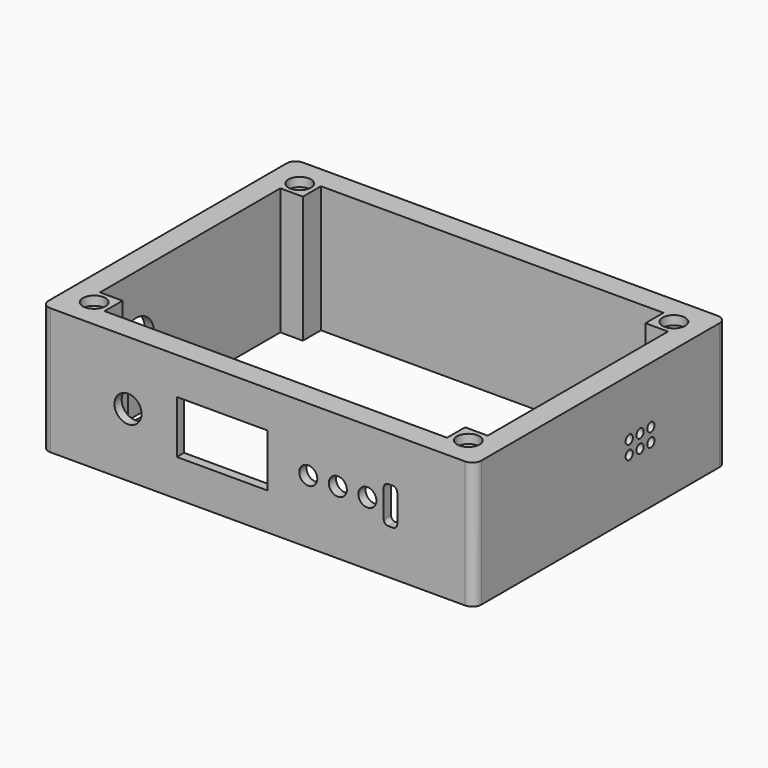
from build123d import *

# Parameters (mm, degrees)
F1_DEPTH  = 28.136
F3_R      = 2.5
F4_DEPTH  = 2
F5_W      = 5
F5_H      = 50
F5_W_2    = 76
F5_H_2    = 5
F6_DEPTH  = 28.137
F7_R      = 1
F8_DEPTH  = 5
F9_R      = 11.25
F9_R_2    = 5
F10_DEPTH = 3
F11_DEPTH = 5
F12_W     = 20.16
F12_H     = 11.72
F12_R     = 3
F12_R_2   = 2
F13_DEPTH = 5
F12_W_2   = 66
F12_H_2   = 18
F12_R_3   = 1.8
F14_DEPTH = 3
F15_DEPTH = 3
F12_R_4   = 0.8
F16_DEPTH = 1.9
F17_DEPTH = 1.9
F18_DEPTH = 1.9
F19_R     = 2.5
F20_DEPTH = 2


# Not quite as in the source:
# - a feature names something its author has since deleted; it is built from what else it names


with BuildPart() as f1:
    # F0 (on Top) → F1 (new body)
    with BuildSketch(Plane.XY):
        with BuildLine():
            Line((46, 35), (-46, 35))
            ThreePointArc((-46, 35), (-47.4142135624, 34.4142135624), (-48, 33))
            Line((-48, 33), (-48, -33))
            ThreePointArc((-48, -33), (-47.4142135624, -34.4142135624), (-46, -35))
            Line((-46, -35), (46, -35))
            ThreePointArc((46, -35), (47.4142135624, -34.4142135624), (48, -33))
            Line((48, -33), (48, 33))
            ThreePointArc((48, 33), (47.4142135624, 34.4142135624), (46, 35))
        make_face()
    extrude(amount=F1_DEPTH)

    # F3 (on face) → F4 (cut)
    with BuildSketch(Plane(origin=(0, 0, 0), x_dir=(1, 0, 0), z_dir=(0, 0, -1))):
        with Locations((-41.5, -28.5)):
            Circle(F3_R)
        with Locations((-41.4999984205, 28.5)):
            Circle(F3_R)
        with Locations((41.5, 28.5)):
            Circle(F3_R)
        with Locations((41.5, -28.5)):
            Circle(F3_R)
    extrude(amount=-F4_DEPTH, mode=Mode.SUBTRACT)

    # F5 (on face) → F6 (cut, through all)
    with BuildSketch(Plane.XY.offset(28.136)):
        with Locations((-40.5, 0)):
            Rectangle(F5_W, F5_H)
        with Locations((0, -27.5)):
            Rectangle(F5_W_2, F5_H_2)
        Rectangle(F5_W_2, F5_H)
        with Locations((0, 27.5)):
            Rectangle(F5_W_2, F5_H_2)
        with Locations((40.5, 0)):
            Rectangle(F5_W, F5_H)
    extrude(amount=-F6_DEPTH, mode=Mode.SUBTRACT)

    # F7 (on face) → F8 (cut, through all)
    with BuildSketch(Plane.YZ.offset(48)):
        with Locations((7.9999985173, 15.568)):
            Circle(F7_R)
        with Locations((7.9999985173, 12.568)):
            Circle(F7_R)
        with Locations((10.9999985173, 12.568)):
            Circle(F7_R)
        with Locations((10.9999985173, 15.568)):
            Circle(F7_R)
        with Locations((13.9999985173, 15.568)):
            Circle(F7_R)
        with Locations((13.9999985173, 12.568)):
            Circle(F7_R)
    extrude(amount=-F8_DEPTH, mode=Mode.SUBTRACT)

    # F9 (on face) → F10 (cut)
    with BuildSketch(Plane(origin=(-48, 0, 0), x_dir=(0, -1, 0), z_dir=(-1, 0, 0))):
        with Locations((15, 14.068)):
            Circle(F9_R)
        with Locations((15, 14.068)):
            Circle(F9_R_2, mode=Mode.SUBTRACT)
    extrude(amount=-F10_DEPTH, mode=Mode.SUBTRACT)

    # F9 (on face) → F11 (cut, through all)
    with BuildSketch(Plane(origin=(-48, 0, 0), x_dir=(0, -1, 0), z_dir=(-1, 0, 0))):
        with Locations((15, 14.068)):
            Circle(F9_R_2)
    extrude(amount=-F11_DEPTH, mode=Mode.SUBTRACT)

    # F12 (on face) → F13 (cut, through all)
    with BuildSketch(Plane(origin=(0, -30, 0), x_dir=(-1, 0, 0), z_dir=(0, 1, 0))):
        with Locations((7.8799169147, 14.0678631142)):
            Rectangle(F12_W, F12_H)
        with Locations((28.7899169147, 14.0678631142)):
            Circle(F12_R)
        with Locations((-11.2000830853, 14.0678631142)):
            Circle(F12_R_2)
        with Locations((-17.7600830853, 14.0678631142)):
            Circle(F12_R_2)
        with Locations((-24.3100830853, 14.0678631142)):
            Circle(F12_R_2)
        with BuildLine():
            ThreePointArc((-30.9400830853, 10.9678631142), (-30.6471898665, 10.260756333), (-29.9400830853, 9.9678631142))
            Line((-29.9400830853, 9.9678631142), (-28.9400830853, 9.9678631142))
            ThreePointArc((-28.9400830853, 9.9678631142), (-28.2329763041, 10.260756333), (-27.9400830853, 10.9678631142))
            Line((-27.9400830853, 10.9678631142), (-27.9400830853, 17.1678631142))
            ThreePointArc((-27.9400830853, 17.1678631142), (-28.2329763041, 17.8749698954), (-28.9400830853, 18.1678631142))
            Line((-28.9400830853, 18.1678631142), (-29.9400830853, 18.1678631142))
            ThreePointArc((-29.9400830853, 18.1678631142), (-30.6471898665, 17.8749698954), (-30.9400830853, 17.1678631142))
            Line((-30.9400830853, 17.1678631142), (-30.9400830853, 10.9678631142))
        make_face()
    extrude(amount=-F13_DEPTH, mode=Mode.SUBTRACT)

    # F12 (on face) → F14 (cut)
    with BuildSketch(Plane(origin=(0, -30, 0), x_dir=(-1, 0, 0), z_dir=(0, 1, 0))):
        with Locations((-0.2100830853, 14.0678631142)):
            Rectangle(F12_W_2, F12_H_2)
        with BuildLine():
            Line((-28.9400830853, 9.9678631142), (-29.9400830853, 9.9678631142))
            ThreePointArc((-29.9400830853, 9.9678631142), (-30.6471898665, 10.260756333), (-30.9400830853, 10.9678631142))
            Line((-30.9400830853, 10.9678631142), (-30.9400830853, 17.1678631142))
            ThreePointArc((-30.9400830853, 17.1678631142), (-30.6471898665, 17.8749698954), (-29.9400830853, 18.1678631142))
            Line((-29.9400830853, 18.1678631142), (-28.9400830853, 18.1678631142))
            ThreePointArc((-28.9400830853, 18.1678631142), (-28.2329763041, 17.8749698954), (-27.9400830853, 17.1678631142))
            Line((-27.9400830853, 17.1678631142), (-27.9400830853, 10.9678631142))
            ThreePointArc((-27.9400830853, 10.9678631142), (-28.2329763041, 10.260756333), (-28.9400830853, 9.9678631142))
        make_face(mode=Mode.SUBTRACT)
        with Locations((-24.3100830853, 14.0678631142)):
            Circle(F12_R_2, mode=Mode.SUBTRACT)
        with Locations((-17.7600830853, 14.0678631142)):
            Circle(F12_R_2, mode=Mode.SUBTRACT)
        with Locations((-11.2000830853, 14.0678631142)):
            Circle(F12_R_2, mode=Mode.SUBTRACT)
        with Locations((7.8799169147, 14.0678631142)):
            Rectangle(F12_W, F12_H, mode=Mode.SUBTRACT)
        with Locations((30.1299169147, 7.5678631142)):
            Circle(F12_R_3, mode=Mode.SUBTRACT)
        with Locations((28.7899169147, 14.0678631142)):
            Circle(F12_R, mode=Mode.SUBTRACT)
        with Locations((-24.0500830853, 20.5678631142)):
            Circle(F12_R_3, mode=Mode.SUBTRACT)
        with Locations((30.1299169147, 20.5678631142)):
            Circle(F12_R_3, mode=Mode.SUBTRACT)
    extrude(amount=F14_DEPTH, mode=Mode.SUBTRACT)

    # F12 (on face) → F15 (cut)
    with BuildSketch(Plane(origin=(0, -30, 0), x_dir=(-1, 0, 0), z_dir=(0, 1, 0))):
        with Locations((-0.2100830853, 14.0678631142)):
            Rectangle(F12_W_2, F12_H_2)
        with BuildLine():
            Line((-28.9400830853, 9.9678631142), (-29.9400830853, 9.9678631142))
            ThreePointArc((-29.9400830853, 9.9678631142), (-30.6471898665, 10.260756333), (-30.9400830853, 10.9678631142))
            Line((-30.9400830853, 10.9678631142), (-30.9400830853, 17.1678631142))
            ThreePointArc((-30.9400830853, 17.1678631142), (-30.6471898665, 17.8749698954), (-29.9400830853, 18.1678631142))
            Line((-29.9400830853, 18.1678631142), (-28.9400830853, 18.1678631142))
            ThreePointArc((-28.9400830853, 18.1678631142), (-28.2329763041, 17.8749698954), (-27.9400830853, 17.1678631142))
            Line((-27.9400830853, 17.1678631142), (-27.9400830853, 10.9678631142))
            ThreePointArc((-27.9400830853, 10.9678631142), (-28.2329763041, 10.260756333), (-28.9400830853, 9.9678631142))
        make_face(mode=Mode.SUBTRACT)
        with Locations((-24.3100830853, 14.0678631142)):
            Circle(F12_R_2, mode=Mode.SUBTRACT)
        with Locations((-17.7600830853, 14.0678631142)):
            Circle(F12_R_2, mode=Mode.SUBTRACT)
        with Locations((-11.2000830853, 14.0678631142)):
            Circle(F12_R_2, mode=Mode.SUBTRACT)
        with Locations((7.8799169147, 14.0678631142)):
            Rectangle(F12_W, F12_H, mode=Mode.SUBTRACT)
        with Locations((30.1299169147, 7.5678631142)):
            Circle(F12_R_3, mode=Mode.SUBTRACT)
        with Locations((28.7899169147, 14.0678631142)):
            Circle(F12_R, mode=Mode.SUBTRACT)
        with Locations((-24.0500830853, 20.5678631142)):
            Circle(F12_R_3, mode=Mode.SUBTRACT)
        with Locations((30.1299169147, 20.5678631142)):
            Circle(F12_R_3, mode=Mode.SUBTRACT)
    extrude(amount=-F15_DEPTH, mode=Mode.SUBTRACT)

    # F12 (on face) → F16 (join)
    with BuildSketch(Plane(origin=(0, -30, 0), x_dir=(-1, 0, 0), z_dir=(0, 1, 0))):
        with Locations((30.1299169147, 20.5678631142)):
            Circle(F12_R_3)
        with Locations((30.1299169147, 20.5678631142)):
            Circle(F12_R_4, mode=Mode.SUBTRACT)
    extrude(amount=F16_DEPTH)

    # F12 (on face) → F17 (join)
    with BuildSketch(Plane(origin=(0, -30, 0), x_dir=(-1, 0, 0), z_dir=(0, 1, 0))):
        with Locations((30.1299169147, 7.5678631142)):
            Circle(F12_R_3)
        with Locations((30.1299169147, 7.5678631142)):
            Circle(F12_R_4, mode=Mode.SUBTRACT)
    extrude(amount=F17_DEPTH)

    # F12 (on face) → F18 (join)
    with BuildSketch(Plane(origin=(0, -30, 0), x_dir=(-1, 0, 0), z_dir=(0, 1, 0))):
        with Locations((-24.0500830853, 20.5678631142)):
            Circle(F12_R_3)
        with Locations((-24.0500830853, 20.5678631142)):
            Circle(F12_R_4, mode=Mode.SUBTRACT)
    extrude(amount=F18_DEPTH)

    # F19 (on face) → F20 (cut)
    with BuildSketch(Plane.XY.offset(28.136)):
        with Locations((-41.5, -28.5)):
            Circle(F19_R)
        with Locations((-41.5, 28.5)):
            Circle(F19_R)
        with Locations((41.5, -28.5)):
            Circle(F19_R)
        with Locations((41.5, 28.5)):
            Circle(F19_R)
    extrude(amount=-F20_DEPTH, mode=Mode.SUBTRACT)


solid = f1.part
